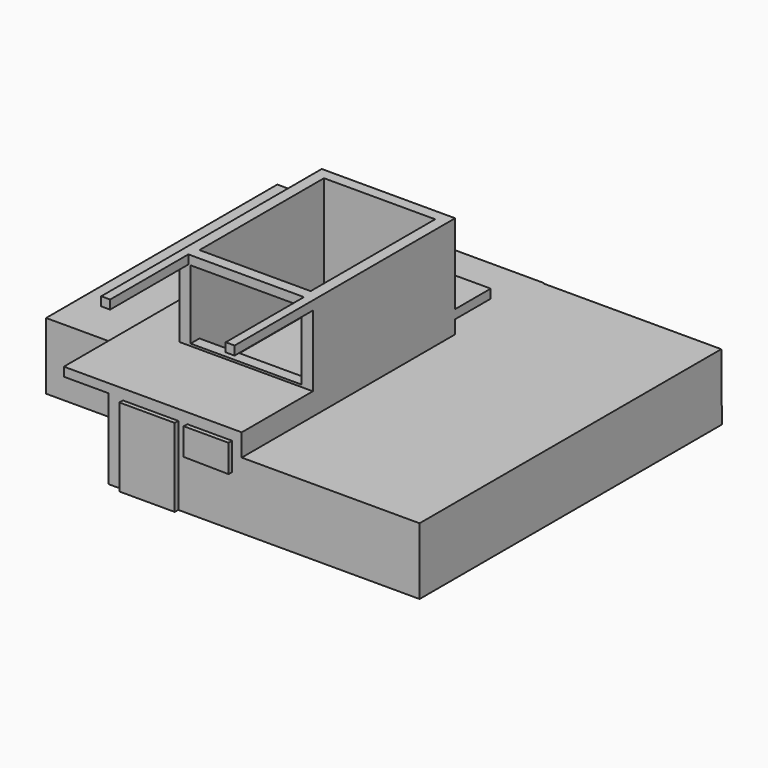
from build123d import *

# Parameters (mm, degrees)
F0_W      = 30
F0_H      = 60
F0_W_2    = 25
F0_H_2    = 55
F1_DEPTH  = 20
F2_W      = 40
F2_H      = 15
F3_DEPTH  = 30
F5_W      = 60
F5_H      = 2
F6_DEPTH  = 10
F8_DEPTH  = 18
F10_DEPTH = 25
F12_DEPTH = 10
F13_W     = 25
F13_H     = 2
F14_DEPTH = 20
F15_W     = 25
F15_H     = 2
F16_DEPTH = 40
F18_DEPTH = 40
F4_W      = 12.4563146383
F4_H      = 17.6308546215
F19_DEPTH = 1
F20_W     = 25
F20_H     = 2.5
F21_DEPTH = 0.5
F22_W     = 2
F22_H     = 2
F23_DEPTH = 22
F26_W     = 2.5
F26_H     = 2
F27_DEPTH = 25


# Not quite as in the source:
# - the program builds the solid bodies; features that only make, move or delete a surface that nothing else refers to are left out


with BuildPart() as f1:
    # F0 (on Top) → F1 (new body)
    with BuildSketch(Plane.XY):
        with Locations((-0.72979182, -0.0160729922)):
            Rectangle(F0_W, F0_H)
        with Locations((-0.72979182, -0.0160729922)):
            Rectangle(F0_W_2, F0_H_2, mode=Mode.SUBTRACT)
    extrude(amount=F1_DEPTH)

    # F2 (on face) → F3 (join)
    with BuildSketch(Plane(origin=(-15.72979182, 0, 0), x_dir=(0, -1, 0), z_dir=(-1, 0, 0))):
        with Locations((-9.9839270078, 7.5)):
            Rectangle(F2_W, F2_H)
    extrude(amount=F3_DEPTH)

    # F5 (on face) → F6 (join)
    with BuildSketch(Plane(origin=(-15.72979182, 0, 0), x_dir=(0, -1, 0), z_dir=(-1, 0, 0))):
        with Locations((0.0160729922, 19)):
            Rectangle(F5_W, F5_H)
    extrude(amount=F6_DEPTH)

    # F7 (on face) → F8 (join)
    with BuildSketch(Plane.XY.offset(20)):
        Polygon((14.27020818, -10.0160729922), (14.27020818, 29.9839270078), (-15.72979182, 29.9839270078), (-15.72979182, -10.0160729922), (-13.22979182, -10.0160729922), (-13.22979182, 27.4839270078), (11.77020818, 27.4839270078), (11.77020818, -10.0160729922), align=None)
    extrude(amount=F8_DEPTH)

    # F9 (on face) → F10 (join)
    with BuildSketch(Plane(origin=(0, 29.9839270078, 0), x_dir=(-1, 0, 0), z_dir=(0, 1, 0))):
        Polygon((45.72979182, 0), (45.72979182, 15), (15.72979182, 15), (-14.27020818, 15), (-14.27020818, 0), align=None)
    extrude(amount=F10_DEPTH)

    # F11 (on face) → F12 (join)
    with BuildSketch(Plane(origin=(0, 29.9839270078, 0), x_dir=(-1, 0, 0), z_dir=(0, 1, 0))):
        Polygon((25.72979182, 18), (25.72979182, 20), (15.72979182, 20), (-14.27020818, 20), (-14.27020818, 18), (15.72979182, 18), align=None)
    extrude(amount=F12_DEPTH)

    # F13 (on face) → F14 (join)
    with BuildSketch(Plane(origin=(0, -27.5160729922, 0), x_dir=(-1, 0, 0), z_dir=(0, 1, 0))):
        with Locations((0.72979182, 19)):
            Rectangle(F13_W, F13_H)
    extrude(amount=F14_DEPTH)

    # F15 (on face) → F16 (join)
    with BuildSketch(Plane.XZ.offset(-27.4839270078)):
        with Locations((-0.72979182, 12)):
            Rectangle(F15_W, F15_H)
    extrude(amount=F16_DEPTH)

    # F17 (on face) → F18 (join)
    with BuildSketch(Plane.YZ.offset(14.27020818)):
        Polygon((54.7944166925, 15), (29.9839270078, 15), (-30.0160729922, 15), (-30.0160729922, 0), (54.9839270078, 0), align=None)
    extrude(amount=F18_DEPTH)

    # F4 (on face) → F19 (join)
    with BuildSketch(Plane.XZ.offset(30.0160729922)):
        with Locations((-6.2281573191, 8.8154273108)):
            Rectangle(F4_W, F4_H)
        Polygon((12.1112056077, 11.4192906767), (12.1112056077, 17.6308546215), (2.0312797278, 17.6308546215), (2.0312797278, 11.5545932204), align=None)
    extrude(amount=F19_DEPTH)

    # F20 (on face) → F21 (join)
    with BuildSketch(Plane.XY.offset(20)):
        with Locations((-0.72979182, -8.7660729922)):
            Rectangle(F20_W, F20_H)
    extrude(amount=F21_DEPTH)

    # F22 (on face) → F23 (join)
    with BuildSketch(Plane.XZ.offset(10.0160729922)):
        with Locations((13.27020818, 37)):
            Rectangle(F22_W, F22_H)
        with Locations((-14.72979182, 37)):
            Rectangle(F22_W, F22_H)
    extrude(amount=F23_DEPTH)

    # F26 (on face) → F27 (join)
    with BuildSketch(Plane(origin=(11.77020818, 0, 0), x_dir=(0, -1, 0), z_dir=(-1, 0, 0))):
        with Locations((8.7660729922, 37)):
            Rectangle(F26_W, F26_H)
    extrude(amount=F27_DEPTH)


solid = f1.part
